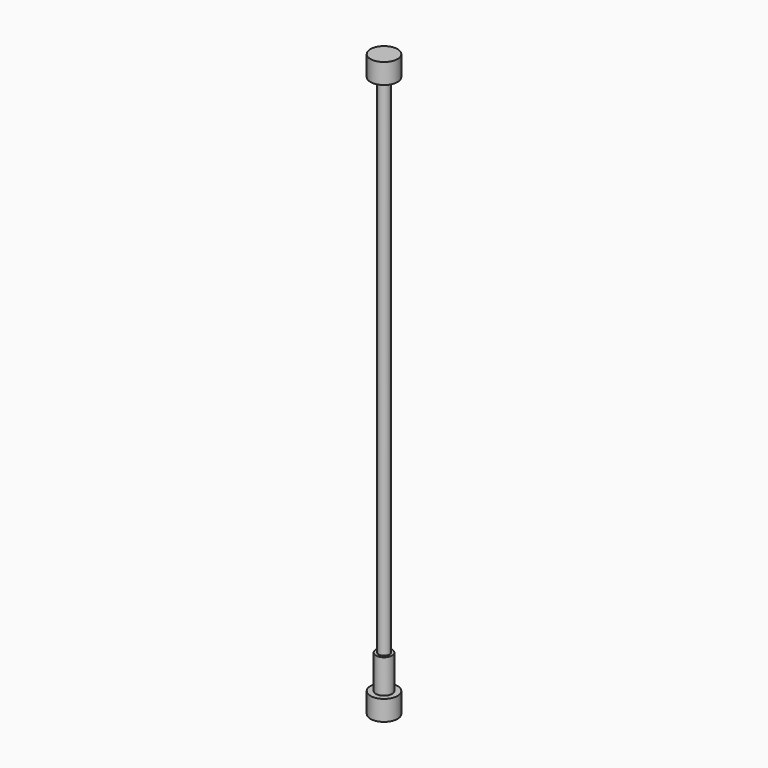
from build123d import *

# Parameters (mm, degrees)
F0_R     = 6
F0_R_2   = 4
F1_DEPTH = 25
F2_R     = 4
F3_DEPTH = 400
F4_R     = 10
F5_DEPTH = 15
F6_R     = 10
F7_DEPTH = 15


with BuildPart() as f1:
    # F0 (on Top) → F1 (new body)
    with BuildSketch(Plane.XY):
        Circle(F0_R)
        Circle(F0_R_2, mode=Mode.SUBTRACT)
    extrude(amount=F1_DEPTH)


with BuildPart() as f3:
    # F2 (on Top) → F3 (new body)
    with BuildSketch(Plane.XY):
        Circle(F2_R)
    extrude(amount=F3_DEPTH)

    # F4 (on face) → F5 (join)
    with BuildSketch(Plane.XY.offset(400)):
        Circle(F4_R)
    extrude(amount=F5_DEPTH)

    # F6 (on face) → F7 (join)
    with BuildSketch(Plane(origin=(0, 0, 0), x_dir=(1, 0, 0), z_dir=(0, 0, -1))):
        Circle(F6_R)
    extrude(amount=F7_DEPTH)


solid = Compound([f1.part, f3.part])
